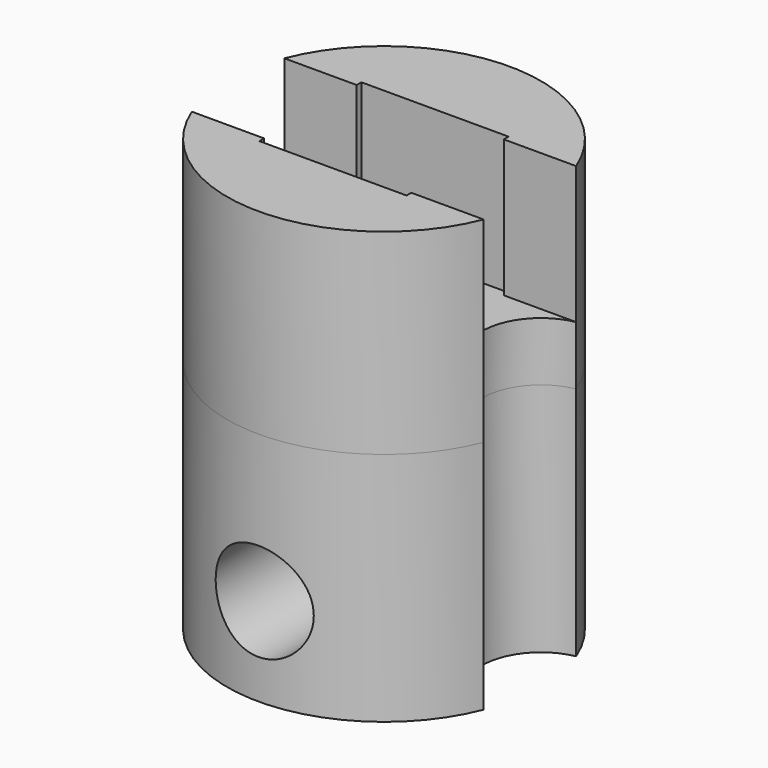
from build123d import *
from build123d import SkipClean  # not in build123d's __all__

# Parameters (mm, degrees)
F0_R           = 8
F1_DEPTH       = 3
F2_R           = 8
F3_DEPTH       = 9
F4_R           = 3
F5_DEPTH       = 12.5
F7_DEPTH       = 10
F8_W           = 4.7
F8_H           = 4.7
F9_DEPTH       = 3
F10_R          = 2.5
F11_DEPTH      = 8.001
F11_DEPTH_BACK = 25


# Not quite as in the source:
# - after a boolean that leaves OpenCascade's solid faulty, fix() repairs it


with BuildPart() as f1:
    # F0 (on Top) → F1 (new body)
    with BuildSketch(Plane.XY):
        Circle(F0_R)
    extrude(amount=F1_DEPTH)

    # F2 (on face) → F3 (join)
    with BuildSketch(Plane(origin=(0, 0, 0), x_dir=(1, 0, 0), z_dir=(0, 0, -1))):
        Circle(F2_R)
    extrude(amount=F3_DEPTH)

    # F4 (on face) → F5 (cut, symmetric)
    with BuildSketch(Plane.XY.offset(3)):
        with Locations((-8, 0)):
            Circle(F4_R)
        with Locations((8, 0)):
            Circle(F4_R)
    extrude(amount=F5_DEPTH, both=True, mode=Mode.SUBTRACT)

    # F6 (on face) → F7 (join)
    with BuildSketch(Plane.XY.offset(3)):
        with BuildLine():
            ThreePointArc((-7.4375, -2.9467938085), (0, -8), (7.4375, -2.9467938085))
            Line((7.4375, -2.9467938085), (3.75, -2.9467938085))
            Line((3.75, -2.9467938085), (3.75, -3.25))
            Line((3.75, -3.25), (-3.75, -3.25))
            Line((-3.75, -3.25), (-3.75, -2.9467938085))
            Line((-3.75, -2.9467938085), (-7.4375, -2.9467938085))
        make_face()
        with BuildLine():
            Line((-3.75, 3.25), (3.75, 3.25))
            Line((3.75, 3.25), (3.75, 2.9467938085))
            Line((3.75, 2.9467938085), (7.4375, 2.9467938085))
            ThreePointArc((7.4375, 2.9467938085), (0, 8), (-7.4375, 2.9467938085))
            Line((-7.4375, 2.9467938085), (-3.75, 2.9467938085))
            Line((-3.75, 2.9467938085), (-3.75, 3.25))
        make_face()
    extrude(amount=F7_DEPTH)

    # F8 (on face) → F9 (join)
    with BuildSketch(Plane.XY.offset(3)):
        with BuildLine():
            ThreePointArc((-7.4375, 2.9467938085), (-5, 0), (-7.4375, -2.9467938085))
            Line((-7.4375, -2.9467938085), (-3.75, -2.9467938085))
            Line((-3.75, -2.9467938085), (-3.75, -3.25))
            Line((-3.75, -3.25), (3.75, -3.25))
            Line((3.75, -3.25), (3.75, -2.9467938085))
            Line((3.75, -2.9467938085), (7.4375, -2.9467938085))
            ThreePointArc((7.4375, -2.9467938085), (5, 0), (7.4375, 2.9467938085))
            Line((7.4375, 2.9467938085), (3.75, 2.9467938085))
            Line((3.75, 2.9467938085), (3.75, 3.25))
            Line((3.75, 3.25), (-3.75, 3.25))
            Line((-3.75, 3.25), (-3.75, 2.9467938085))
            Line((-3.75, 2.9467938085), (-7.4375, 2.9467938085))
        make_face()
        Rectangle(F8_W, F8_H, mode=Mode.SUBTRACT)
    with SkipClean():  # cleaning this boolean's faces spoils the solid; the shape is the same uncleaned
        extrude(amount=F9_DEPTH)

    # F10 (on Front) → F11 (cut, two sides)
    with BuildSketch(Plane.XZ) as f11_sk:
        with Locations((0, -4.5)):
            Circle(F10_R)
    extrude(amount=-F11_DEPTH, mode=Mode.SUBTRACT)
    extrude(f11_sk.sketch, amount=F11_DEPTH_BACK, mode=Mode.SUBTRACT)

    add(f1.part.fix(), mode=Mode.REPLACE)


solid = f1.part
